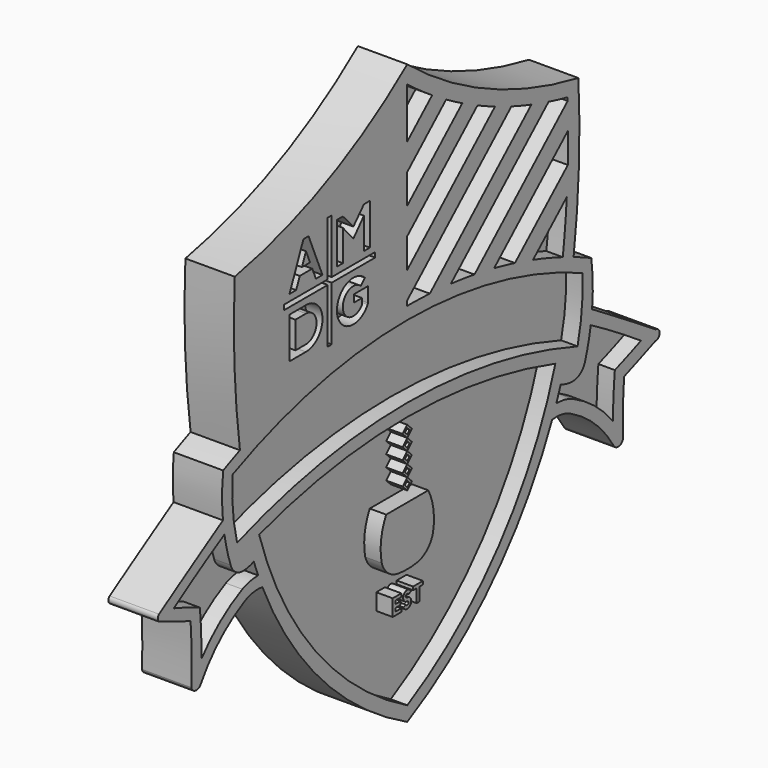
from build123d import *

# Parameters (mm, degrees)
F2_DEPTH = 7.62
F3_DEPTH = 5.08
F4_DEPTH = 7.62


# Not quite as in the source:
# - a feature names something its author has since deleted; it is built from what else it names


with BuildPart() as f2:
    # F0 (on Right) → F2 (new body)
    with BuildSketch(Plane.YZ):
        with BuildLine():
            ThreePointArc((28.5688662104, -6.671875786), (17.7209639174, -26.8909401666), (0, -41.4667758689))
            Line((0, -41.4667758689), (0, -43.7257877909))
            ThreePointArc((0, -43.7257877909), (16.5196456669, -31.2816632656), (27.9511640539, -14.0457903394))
            ThreePointArc((27.9511640539, -14.0457903394), (28.3611811829, -13.0956454783), (28.7550746015, -12.1387038511))
            ThreePointArc((28.7550746015, -12.1387038511), (29.189869611, -11.0251738196), (29.6028329723, -9.9033640792))
            ThreePointArc((29.6028329723, -9.9033640792), (30.0512558711, -8.6014682185), (30.4702761414, -7.2898135606))
            ThreePointArc((30.4702761414, -7.2898135606), (29.5211880551, -6.9758694959), (28.5688662104, -6.671875786))
        make_face()
        with BuildLine():
            ThreePointArc((-29.6028329723, -9.9033640792), (-30.0512558711, -8.6014682185), (-30.4702761414, -7.2898135606))
            ThreePointArc((-30.4702761414, -7.2898135606), (-32.275717496, -7.9177084152), (-34.0682319546, -8.5816077668))
            ThreePointArc((-34.0682319546, -8.5816077668), (-33.1727263346, -9.8516485544), (-31.6970650168, -10.3388421429))
            ThreePointArc((-31.6970650168, -10.3388421429), (-30.6278933435, -10.2271696504), (-29.6028329723, -9.9033640792))
        make_face()
        with BuildLine():
            ThreePointArc((34.3090759298, -8.673933633), (32.3970687067, -7.9613703293), (30.4702761414, -7.2898135606))
            ThreePointArc((30.4702761414, -7.2898135606), (30.0512558711, -8.6014682185), (29.6028329723, -9.9033640792))
            ThreePointArc((29.6028329723, -9.9033640792), (30.7403743709, -10.2999751342), (31.9379090014, -10.4311680127))
            ThreePointArc((31.9379090014, -10.4311680127), (33.4135703165, -9.9439744228), (34.3090759298, -8.673933633))
        make_face()
        with BuildLine():
            ThreePointArc((28.7550746015, -12.1387038511), (28.3611811829, -13.0956454783), (27.9511640539, -14.0457903394))
            ThreePointArc((27.9511640539, -14.0457903394), (29.8035313011, -14.0664319634), (31.5502868159, -14.6833076938))
            ThreePointArc((31.5502868159, -14.6833076938), (36.1922706404, -17.9362667961), (39.7833809257, -22.321889177))
            ThreePointArc((39.7833809257, -22.321889177), (40.7955153713, -22.88098694), (41.6602343321, -22.1133492887))
            ThreePointArc((41.6602343321, -22.1133492887), (41.6260167095, -17.9626931556), (41.8306558255, -13.8169435234))
            ThreePointArc((41.8306558255, -13.8169435234), (44.8619911882, -12.6385051681), (47.8847744868, -11.4383001158))
            ThreePointArc((47.8847744868, -11.4383001158), (48.6831556004, -10.6892682312), (47.9341237159, -9.8908871176))
            ThreePointArc((47.9341237159, -9.8908871176), (41.8140573783, -5.9988864798), (35.658738053, -2.1628827072))
            ThreePointArc((35.658738053, -2.1628827072), (35.5441808227, -3.1869322299), (35.394852187, -4.2064918125))
            ThreePointArc((35.394852187, -4.2064918125), (40.2885281884, -7.1486484466), (45.0794595538, -10.25530696))
            ThreePointArc((45.0794595538, -10.25530696), (42.5737442672, -11.2633717283), (40.041684099, -12.2033052254))
            ThreePointArc((40.041684099, -12.2033052254), (39.7867159057, -15.5987236175), (39.68812496, -19.0022739201))
            ThreePointArc((39.68812496, -19.0022739201), (36.1022922808, -15.4419861489), (31.8168029189, -12.7645945176))
            ThreePointArc((31.8168029189, -12.7645945176), (30.3188612648, -12.2905990682), (28.7550746015, -12.1387038511))
        make_face()
        with BuildLine():
            ThreePointArc((-27.9511640539, -14.0457903394), (-28.3611811829, -13.0956454783), (-28.7550746015, -12.1387038511))
            ThreePointArc((-28.7550746015, -12.1387038511), (-30.3188612648, -12.2905990682), (-31.8168029189, -12.7645945176))
            ThreePointArc((-31.8168029189, -12.7645945176), (-36.1022922808, -15.4419861489), (-39.68812496, -19.0022739201))
            ThreePointArc((-39.68812496, -19.0022739201), (-39.7567496729, -15.4652900802), (-39.9942449201, -11.9356215344))
            ThreePointArc((-39.9942449201, -11.9356215344), (-42.4943140259, -10.9129550124), (-45.0320203748, -9.987623269))
            ThreePointArc((-45.0320203748, -9.987623269), (-40.2016909636, -6.8727936195), (-35.2677039574, -3.9249099398))
            ThreePointArc((-35.2677039574, -3.9249099398), (-35.4270693541, -2.9093430207), (-35.5518756641, -1.8889524672))
            ThreePointArc((-35.5518756641, -1.8889524672), (-41.7369860787, -5.7278399379), (-47.8866845382, -9.6232034266))
            ThreePointArc((-47.8866845382, -9.6232034266), (-48.1257262457, -10.1509293815), (-47.8520728648, -10.6615656987))
            ThreePointArc((-47.8520728648, -10.6615656987), (-44.8292895661, -11.861770751), (-41.7979542035, -13.0402091063))
            ThreePointArc((-41.7979542035, -13.0402091063), (-41.5863132676, -17.5746119455), (-41.6602343321, -22.1133492887))
            ThreePointArc((-41.6602343321, -22.1133492887), (-40.7955153713, -22.88098694), (-39.7833809257, -22.321889177))
            ThreePointArc((-39.7833809257, -22.321889177), (-36.1922706404, -17.9362667961), (-31.5502868159, -14.6833076938))
            ThreePointArc((-31.5502868159, -14.6833076938), (-29.8035313011, -14.0664319634), (-27.9511640539, -14.0457903394))
        make_face()
        with BuildLine():
            ThreePointArc((-28.5688662104, -6.671875786), (-29.5211880551, -6.9758694959), (-30.4702761414, -7.2898135606))
            ThreePointArc((-30.4702761414, -7.2898135606), (-30.0512558711, -8.6014682185), (-29.6028329723, -9.9033640792))
            ThreePointArc((-29.6028329723, -9.9033640792), (-29.189869611, -11.0251738196), (-28.7550746015, -12.1387038511))
            ThreePointArc((-28.7550746015, -12.1387038511), (-28.3611811829, -13.0956454783), (-27.9511640539, -14.0457903394))
            ThreePointArc((-27.9511640539, -14.0457903394), (-16.5196456669, -31.2816632656), (0, -43.7257877909))
            Line((0, -43.7257877909), (0, -41.4667758689))
            ThreePointArc((0, -41.4667758689), (-17.7209639174, -26.8909401666), (-28.5688662104, -6.671875786))
        make_face()
        with BuildLine():
            ThreePointArc((-34.0682319546, -8.5816077668), (-32.275717496, -7.9177084152), (-30.4702761414, -7.2898135606))
            ThreePointArc((-30.4702761414, -7.2898135606), (-29.5211880551, -6.9758694959), (-28.5688662104, -6.671875786))
            ThreePointArc((-28.5688662104, -6.671875786), (0, -2.299220842), (28.5688662104, -6.671875786))
            ThreePointArc((28.5688662104, -6.671875786), (29.5211880551, -6.9758694959), (30.4702761414, -7.2898135606))
            ThreePointArc((30.4702761414, -7.2898135606), (32.3970687067, -7.9613703293), (34.3090759298, -8.673933633))
            ThreePointArc((34.3090759298, -8.673933633), (34.9368600064, -6.4608460088), (35.394852187, -4.2064918125))
            ThreePointArc((35.394852187, -4.2064918125), (35.5441808227, -3.1869322299), (35.658738053, -2.1628827072))
            ThreePointArc((35.658738053, -2.1628827072), (35.7862431554, 1.3568364417), (35.5042511946, 4.8675573039))
            ThreePointArc((35.5042511946, 4.8675573039), (33.8050800577, 5.643593937), (32.088958966, 6.3813905261))
            ThreePointArc((32.088958966, 6.3813905261), (31.0516229156, 6.805512456), (30.008682983, 7.2156609533))
            ThreePointArc((30.008682983, 7.2156609533), (27.1584492935, 8.2553731736), (24.2722940751, 9.1907563256))
            ThreePointArc((24.2722940751, 9.1907563256), (22.5250389094, 9.7013614162), (20.7670586297, 10.1737209285))
            ThreePointArc((20.7670586297, 10.1737209285), (18.7644701082, 10.6621519958), (16.7504251557, 11.100955623))
            ThreePointArc((16.7504251557, 11.100955623), (14.8629765183, 11.4652081673), (12.9676361757, 11.7858750662))
            ThreePointArc((12.9676361757, 11.7858750662), (10.6902549144, 12.1121256668), (8.4047431756, 12.3754523754))
            ThreePointArc((8.4047431756, 12.3754523754), (6.3842218408, 12.5552704602), (4.3599256973, 12.6859078666))
            ThreePointArc((4.3599256973, 12.6859078666), (2.180708045, 12.7714103093), (0, 12.799917618))
            ThreePointArc((0, 12.799917618), (-16.4600536871, 11.15993435), (-32.2729385148, 6.3044646579))
            ThreePointArc((-32.2729385148, 6.3044646579), (-33.8962097721, 5.6031353828), (-35.5042511946, 4.8675573039))
            ThreePointArc((-35.5042511946, 4.8675573039), (-35.7170770288, 1.4906347145), (-35.5518756641, -1.8889524672))
            ThreePointArc((-35.5518756641, -1.8889524672), (-35.4270693541, -2.9093430207), (-35.2677039574, -3.9249099398))
            ThreePointArc((-35.2677039574, -3.9249099398), (-34.7605382134, -6.2771030958), (-34.0682319546, -8.5816077668))
        make_face()
        with BuildLine():
            ThreePointArc((-33.7083284733, 3.5726207659), (-17.2446774523, 9.025399368), (0, 10.8708529679))
            ThreePointArc((0, 10.8708529679), (17.2896098342, 9.0156577322), (33.792024647, 3.5345389662))
            ThreePointArc((33.792024647, 3.5345389662), (33.6890042384, -1.2985833574), (32.8517336285, -6.0597452457))
            ThreePointArc((32.8517336285, -6.0597452457), (0.0193967345, -0.3558691534), (-32.8152080177, -6.0466757012))
            ThreePointArc((-32.8152080177, -6.0466757012), (-33.6517360253, -1.2732347103), (-33.7083284733, 3.5726207659))
        make_face(mode=Mode.SUBTRACT)
        with BuildLine():
            ThreePointArc((-33.2703815176, 30.2840155791), (-33.3383945489, 18.2706664746), (-32.2729385148, 6.3044646579))
            ThreePointArc((-32.2729385148, 6.3044646579), (-16.4600536871, 11.15993435), (0, 12.799917618))
            Line((0, 12.799917618), (0, 13.5470115411))
            Line((0, 13.5470115411), (0, 17.6854213957))
            Line((0, 17.6854213957), (0, 22.2660372864))
            Line((0, 22.2660372864), (0, 26.4044471422))
            Line((0, 26.4044471422), (0, 30.9850630336))
            Line((0, 30.9850630336), (0, 35.123472889))
            Line((0, 35.123472889), (0, 42.8770001444))
            ThreePointArc((0, 42.8770001444), (2.3677216766, 41.1256679461), (4.8004917628, 39.4658787684))
            ThreePointArc((4.8004917628, 39.4658787684), (6.1440586372, 38.6059679212), (7.5050988374, 37.7739894453))
            ThreePointArc((7.5050988374, 37.7739894453), (9.0521255608, 36.8742809791), (10.619583518, 36.0106592104))
            ThreePointArc((10.619583518, 36.0106592104), (12.0755875899, 35.2501172378), (13.5474374931, 34.5207135003))
            ThreePointArc((13.5474374931, 34.5207135003), (15.2251273318, 33.736066262), (16.9211499837, 32.9918743189))
            ThreePointArc((16.9211499837, 32.9918743189), (18.5018678165, 32.3413130995), (20.0965961968, 31.7258944125))
            ThreePointArc((20.0965961968, 31.7258944125), (22.0128328658, 31.0392961839), (23.9464982844, 30.4034360204))
            ThreePointArc((23.9464982844, 30.4034360204), (25.6026977209, 29.9032123795), (27.2696864447, 29.4402125321))
            ThreePointArc((27.2696864447, 29.4402125321), (29.09371693, 28.979244413), (30.9284345114, 28.5628429071))
            ThreePointArc((30.9284345114, 28.5628429071), (30.9390866234, 28.3072147129), (30.94921453, 28.0515652133))
            ThreePointArc((30.94921453, 28.0515652133), (31.0106105135, 26.039411949), (31.0395347413, 24.0265300312))
            ThreePointArc((31.0395347413, 24.0265300312), (31.0323022412, 21.6837727985), (30.9810838152, 19.3415643464))
            ThreePointArc((30.9810838152, 19.3415643464), (30.8960102432, 17.2060844583), (30.7743721396, 15.0723750036))
            ThreePointArc((30.7743721396, 15.0723750036), (30.4536777009, 11.1379610331), (30.008682983, 7.2156609533))
            ThreePointArc((30.008682983, 7.2156609533), (31.0516229156, 6.805512456), (32.088958966, 6.3813905261))
            ThreePointArc((32.088958966, 6.3813905261), (33.1186305942, 18.334974947), (33.0151768056, 30.3323788948))
            ThreePointArc((33.0151768056, 30.3323788948), (15.5682047755, 35.9423036807), (0, 45.6117963866))
            ThreePointArc((0, 45.6117963866), (-15.7054175834, 35.9297463642), (-33.2703815176, 30.2840155791))
        make_face()
        with BuildLine():
            Line((-22.7114348597, 14.4936506769), (-22.7114348597, 20.8402629143))
            Line((-22.7114348597, 20.8402629143), (-19.5476338267, 20.8402629143))
            ThreePointArc((-19.5476338267, 20.8402629143), (-16.3508674463, 17.6669567956), (-19.5476338267, 14.4936506769))
            Line((-19.5476338267, 14.4936506769), (-22.7114348597, 14.4936506769))
        make_face(mode=Mode.SUBTRACT)
        Polygon((-6.189193825, 21.8708057269), (-14.578833418, 21.8708057269), (-14.578833418, 13.4811661339), (-15.3361896718, 13.4811661339), (-15.3361896718, 21.8708057269), (-23.7258292649, 21.8708057269), (-23.7258292649, 22.6281619807), (-15.3361896718, 22.6281619807), (-15.3361896718, 31.0178015738), (-14.578833418, 31.0178015738), (-14.578833418, 22.6281619807), (-6.189193825, 22.6281619807), align=None, mode=Mode.SUBTRACT)
        with BuildLine():
            Line((-8.1508552757, 19.9294396921), (-8.9558750817, 19.1224107936))
            ThreePointArc((-8.9558750817, 19.1224107936), (-12.4318439094, 17.5698783849), (-8.8166163828, 16.3770472559))
            ThreePointArc((-8.8166163828, 16.3770472559), (-8.7538836126, 16.4763115742), (-8.7319527365, 16.5916711946))
            Line((-8.7319527365, 16.5916711946), (-8.7319527365, 17.4191270619))
            Line((-8.7319527365, 17.4191270619), (-10.3048576847, 17.4191270619))
            Line((-10.3048576847, 17.4191270619), (-10.3058647235, 18.5571518939))
            Line((-10.3058647235, 18.5571518939), (-7.5927416105, 18.5595527382))
            Line((-7.5927416105, 18.5595527382), (-7.590726548, 16.2823902296))
            ThreePointArc((-7.590726548, 16.2823902296), (-7.6034442607, 16.178744507), (-7.6410153285, 16.0813145788))
            ThreePointArc((-7.6410153285, 16.0813145788), (-13.5400716848, 17.2575827913), (-8.1508552757, 19.9294396921))
        make_face(mode=Mode.SUBTRACT)
        Polygon((-20.0286190957, 29.9993950033), (-19.0364969938, 29.9993950033), (-16.3545962423, 23.6434713984), (-17.6239740103, 23.6434713984), (-18.3205924604, 25.2944100648), (-20.7354008474, 25.2944100648), (-21.4320192974, 23.6434713984), (-22.7105198472, 23.6434713984), align=None, mode=Mode.SUBTRACT)
        Polygon((-12.4187339097, 28.4452587366), (-12.4187339097, 23.6434713984), (-13.5635240003, 23.6434713984), (-13.5635240003, 29.9993950033), (-12.4187339097, 29.9993950033), (-10.3889470469, 27.789356187), (-8.359160184, 29.9993950033), (-7.2075975113, 29.9993950033), (-7.2075975113, 23.6386322463), (-8.359160184, 23.6386322463), (-8.359160184, 28.4452587366), (-10.3889470469, 26.1637270451), align=None, mode=Mode.SUBTRACT)
        with BuildLine():
            Line((0, 35.123472889), (0, 30.9850630336))
            Line((0, 30.9850630336), (7.5050988374, 37.7739894453))
            ThreePointArc((7.5050988374, 37.7739894453), (6.1440586372, 38.6059679212), (4.8004917628, 39.4658787684))
            Line((4.8004917628, 39.4658787684), (0, 35.123472889))
        make_face()
        with BuildLine():
            Line((0, 26.4044471422), (0, 22.2660372864))
            Line((0, 22.2660372864), (13.5474374931, 34.5207135003))
            ThreePointArc((13.5474374931, 34.5207135003), (12.0755875899, 35.2501172378), (10.619583518, 36.0106592104))
            Line((10.619583518, 36.0106592104), (0, 26.4044471422))
        make_face()
        with BuildLine():
            Line((0, 17.6854213957), (0, 13.5470115411))
            Line((0, 13.5470115411), (20.0965961968, 31.7258944125))
            ThreePointArc((20.0965961968, 31.7258944125), (18.5018678165, 32.3413130995), (16.9211499837, 32.9918743189))
            Line((16.9211499837, 32.9918743189), (0, 17.6854213957))
        make_face()
        with BuildLine():
            Line((23.9464982844, 30.4034360204), (4.3599256973, 12.6859078666))
            ThreePointArc((4.3599256973, 12.6859078666), (6.3842218408, 12.5552704602), (8.4047431756, 12.3754523754))
            Line((8.4047431756, 12.3754523754), (27.2696864447, 29.4402125321))
            ThreePointArc((27.2696864447, 29.4402125321), (25.6026977209, 29.9032123795), (23.9464982844, 30.4034360204))
        make_face()
        with BuildLine():
            Line((30.94921453, 28.0515652133), (12.9676361757, 11.7858750662))
            ThreePointArc((12.9676361757, 11.7858750662), (14.8629765183, 11.4652081673), (16.7504251557, 11.100955623))
            Line((16.7504251557, 11.100955623), (31.0395347413, 24.0265300312))
            ThreePointArc((31.0395347413, 24.0265300312), (31.0106105135, 26.039411949), (30.94921453, 28.0515652133))
        make_face()
        with BuildLine():
            ThreePointArc((20.7670586297, 10.1737209285), (22.5250389094, 9.7013614162), (24.2722940751, 9.1907563256))
            Line((24.2722940751, 9.1907563256), (30.7743721396, 15.0723750036))
            ThreePointArc((30.7743721396, 15.0723750036), (30.8960102432, 17.2060844583), (30.9810838152, 19.3415643464))
            Line((30.9810838152, 19.3415643464), (20.7670586297, 10.1737209285))
        make_face()
    extrude(amount=F2_DEPTH)


with BuildPart() as f2b:
    # F0 (on Right) → F2, piece 2 (new body)
    with BuildSketch(Plane.YZ):
        Polygon((-19.5279966539, 28.1558764371), (-20.3060973907, 26.3118302556), (-18.7498959171, 26.3118302556), align=None)
    extrude(amount=F2_DEPTH)


with BuildPart() as f2c:
    # F0 (on Right) → F2, piece 3 (new body)
    with BuildSketch(Plane.YZ):
        with BuildLine():
            Line((-21.5756800026, 19.6895375848), (-21.5756800026, 15.5159393325))
            Line((-21.5756800026, 15.5159393325), (-19.5476338267, 15.5159393325))
            ThreePointArc((-19.5476338267, 15.5159393325), (-17.4972787499, 17.6027384587), (-19.5476338267, 19.6895375848))
            Line((-19.5476338267, 19.6895375848), (-21.5756800026, 19.6895375848))
        make_face()
    extrude(amount=F2_DEPTH)


with BuildPart() as f3:
    # F0 (on Right) → F3 (new body)
    with BuildSketch(Plane.YZ):
        with BuildLine():
            ThreePointArc((33.792024647, 3.5345389662), (17.2896098342, 9.0156577322), (0, 10.8708529679))
            ThreePointArc((0, 10.8708529679), (-17.2446774523, 9.025399368), (-33.7083284733, 3.5726207659))
            ThreePointArc((-33.7083284733, 3.5726207659), (-33.6517360253, -1.2732347103), (-32.8152080177, -6.0466757012))
            ThreePointArc((-32.8152080177, -6.0466757012), (0.0193967345, -0.3558691534), (32.8517336285, -6.0597452457))
            ThreePointArc((32.8517336285, -6.0597452457), (33.6890042384, -1.2985833574), (33.792024647, 3.5345389662))
        make_face()
    extrude(amount=F3_DEPTH)


with BuildPart() as f3b:
    # F0 (on Right) → F3, piece 2 (new body)
    with BuildSketch(Plane.YZ):
        with BuildLine():
            ThreePointArc((28.5688662104, -6.671875786), (0, -2.299220842), (-28.5688662104, -6.671875786))
            ThreePointArc((-28.5688662104, -6.671875786), (-17.7209639174, -26.8909401666), (0, -41.4667758689))
            ThreePointArc((0, -41.4667758689), (17.7209639174, -26.8909401666), (28.5688662104, -6.671875786))
        make_face()
    extrude(amount=F3_DEPTH)


with BuildPart() as f3c:
    # F0 (on Right) → F3, piece 3 (new body)
    with BuildSketch(Plane.YZ):
        Polygon((-13.5635240003, 23.6434713984), (-12.4187339097, 23.6434713984), (-12.4187339097, 28.4452587366), (-10.3889470469, 26.1637270451), (-8.359160184, 28.4452587366), (-8.359160184, 23.6386322463), (-7.2075975113, 23.6386322463), (-7.2075975113, 29.9993950033), (-8.359160184, 29.9993950033), (-10.3889470469, 27.789356187), (-12.4187339097, 29.9993950033), (-13.5635240003, 29.9993950033), align=None)
    extrude(amount=F3_DEPTH)


with BuildPart() as f3d:
    # F0 (on Right) → F3, piece 4 (new body)
    with BuildSketch(Plane.YZ):
        Polygon((-16.3545962423, 23.6434713984), (-19.0364969938, 29.9993950033), (-20.0286190957, 29.9993950033), (-22.7105198472, 23.6434713984), (-21.4320192974, 23.6434713984), (-20.7354008474, 25.2944100648), (-18.3205924604, 25.2944100648), (-17.6239740103, 23.6434713984), align=None)
        Polygon((-18.7498959171, 26.3118302556), (-20.3060973907, 26.3118302556), (-19.5279966539, 28.1558764371), align=None, mode=Mode.SUBTRACT)
    extrude(amount=F3_DEPTH)


with BuildPart() as f3e:
    # F0 (on Right) → F3, piece 5 (new body)
    with BuildSketch(Plane.YZ):
        with BuildLine():
            Line((-19.5476338267, 20.8402629143), (-22.7114348597, 20.8402629143))
            Line((-22.7114348597, 20.8402629143), (-22.7114348597, 14.4936506769))
            Line((-22.7114348597, 14.4936506769), (-19.5476338267, 14.4936506769))
            ThreePointArc((-19.5476338267, 14.4936506769), (-16.3508674463, 17.6669567956), (-19.5476338267, 20.8402629143))
        make_face()
        with BuildLine():
            Line((-19.5476338267, 15.5159393325), (-21.5756800026, 15.5159393325))
            Line((-21.5756800026, 15.5159393325), (-21.5756800026, 19.6895375848))
            Line((-21.5756800026, 19.6895375848), (-19.5476338267, 19.6895375848))
            ThreePointArc((-19.5476338267, 19.6895375848), (-17.4972787499, 17.6027384587), (-19.5476338267, 15.5159393325))
        make_face(mode=Mode.SUBTRACT)
    extrude(amount=F3_DEPTH)


with BuildPart() as f3f:
    # F0 (on Right) → F3, piece 6 (new body)
    with BuildSketch(Plane.YZ):
        Polygon((-14.578833418, 13.4811661339), (-14.578833418, 21.8708057269), (-6.189193825, 21.8708057269), (-6.189193825, 22.6281619807), (-14.578833418, 22.6281619807), (-14.578833418, 31.0178015738), (-15.3361896718, 31.0178015738), (-15.3361896718, 22.6281619807), (-23.7258292649, 22.6281619807), (-23.7258292649, 21.8708057269), (-15.3361896718, 21.8708057269), (-15.3361896718, 13.4811661339), align=None)
    extrude(amount=F3_DEPTH)


with BuildPart() as f3g:
    # F0 (on Right) → F3, piece 7 (new body)
    with BuildSketch(Plane.YZ):
        with BuildLine():
            ThreePointArc((31.9379090014, -10.4311680127), (30.7403743709, -10.2999751342), (29.6028329723, -9.9033640792))
            ThreePointArc((29.6028329723, -9.9033640792), (29.189869611, -11.0251738196), (28.7550746015, -12.1387038511))
            ThreePointArc((28.7550746015, -12.1387038511), (30.3188612648, -12.2905990682), (31.8168029189, -12.7645945176))
            ThreePointArc((31.8168029189, -12.7645945176), (36.1022922808, -15.4419861489), (39.68812496, -19.0022739201))
            ThreePointArc((39.68812496, -19.0022739201), (39.7867159057, -15.5987236175), (40.041684099, -12.2033052254))
            ThreePointArc((40.041684099, -12.2033052254), (42.5737442672, -11.2633717283), (45.0794595538, -10.25530696))
            ThreePointArc((45.0794595538, -10.25530696), (40.2885281884, -7.1486484466), (35.394852187, -4.2064918125))
            ThreePointArc((35.394852187, -4.2064918125), (34.9368600064, -6.4608460088), (34.3090759298, -8.673933633))
            ThreePointArc((34.3090759298, -8.673933633), (33.4135703165, -9.9439744228), (31.9379090014, -10.4311680127))
        make_face()
    extrude(amount=F3_DEPTH)


with BuildPart() as f3h:
    # F0 (on Right) → F3, piece 8 (new body)
    with BuildSketch(Plane.YZ):
        with BuildLine():
            ThreePointArc((-28.7550746015, -12.1387038511), (-29.189869611, -11.0251738196), (-29.6028329723, -9.9033640792))
            ThreePointArc((-29.6028329723, -9.9033640792), (-30.6278933435, -10.2271696504), (-31.6970650168, -10.3388421429))
            ThreePointArc((-31.6970650168, -10.3388421429), (-33.1727263346, -9.8516485544), (-34.0682319546, -8.5816077668))
            ThreePointArc((-34.0682319546, -8.5816077668), (-34.7605382134, -6.2771030958), (-35.2677039574, -3.9249099398))
            ThreePointArc((-35.2677039574, -3.9249099398), (-40.2016909636, -6.8727936195), (-45.0320203748, -9.987623269))
            ThreePointArc((-45.0320203748, -9.987623269), (-42.4943140259, -10.9129550124), (-39.9942449201, -11.9356215344))
            ThreePointArc((-39.9942449201, -11.9356215344), (-39.7567496729, -15.4652900802), (-39.68812496, -19.0022739201))
            ThreePointArc((-39.68812496, -19.0022739201), (-36.1022922808, -15.4419861489), (-31.8168029189, -12.7645945176))
            ThreePointArc((-31.8168029189, -12.7645945176), (-30.3188612648, -12.2905990682), (-28.7550746015, -12.1387038511))
        make_face()
    extrude(amount=F3_DEPTH)


with BuildPart() as f3i:
    # F0 (on Right) → F3, piece 9 (new body)
    with BuildSketch(Plane.YZ):
        with BuildLine():
            ThreePointArc((-8.8166163828, 16.3770472559), (-12.4318439094, 17.5698783849), (-8.9558750817, 19.1224107936))
            Line((-8.9558750817, 19.1224107936), (-8.1508552757, 19.9294396921))
            ThreePointArc((-8.1508552757, 19.9294396921), (-13.5400716848, 17.2575827913), (-7.6410153285, 16.0813145788))
            ThreePointArc((-7.6410153285, 16.0813145788), (-7.6034442607, 16.178744507), (-7.590726548, 16.2823902296))
            Line((-7.590726548, 16.2823902296), (-7.5927416105, 18.5595527382))
            Line((-7.5927416105, 18.5595527382), (-10.3058647235, 18.5571518939))
            Line((-10.3058647235, 18.5571518939), (-10.3048576847, 17.4191270619))
            Line((-10.3048576847, 17.4191270619), (-8.7319527365, 17.4191270619))
            Line((-8.7319527365, 17.4191270619), (-8.7319527365, 16.5916711946))
            ThreePointArc((-8.7319527365, 16.5916711946), (-8.7538836126, 16.4763115742), (-8.8166163828, 16.3770472559))
        make_face()
    extrude(amount=F3_DEPTH)


with BuildPart() as f3j:
    # F0 (on Right) → F3, piece 10 (new body)
    with BuildSketch(Plane.YZ):
        with BuildLine():
            Line((0, 42.8770001444), (0, 35.123472889))
            Line((0, 35.123472889), (4.8004917628, 39.4658787684))
            ThreePointArc((4.8004917628, 39.4658787684), (2.3677216766, 41.1256679461), (0, 42.8770001444))
        make_face()
    extrude(amount=F3_DEPTH)


with BuildPart() as f3k:
    # F0 (on Right) → F3, piece 11 (new body)
    with BuildSketch(Plane.YZ):
        with BuildLine():
            Line((0, 30.9850630336), (0, 26.4044471422))
            Line((0, 26.4044471422), (10.619583518, 36.0106592104))
            ThreePointArc((10.619583518, 36.0106592104), (9.0521255608, 36.8742809791), (7.5050988374, 37.7739894453))
            Line((7.5050988374, 37.7739894453), (0, 30.9850630336))
        make_face()
    extrude(amount=F3_DEPTH)


with BuildPart() as f3l:
    # F0 (on Right) → F3, piece 12 (new body)
    with BuildSketch(Plane.YZ):
        with BuildLine():
            Line((0, 22.2660372864), (0, 17.6854213957))
            Line((0, 17.6854213957), (16.9211499837, 32.9918743189))
            ThreePointArc((16.9211499837, 32.9918743189), (15.2251273318, 33.736066262), (13.5474374931, 34.5207135003))
            Line((13.5474374931, 34.5207135003), (0, 22.2660372864))
        make_face()
    extrude(amount=F3_DEPTH)


with BuildPart() as f3m:
    # F0 (on Right) → F3, piece 13 (new body)
    with BuildSketch(Plane.YZ):
        with BuildLine():
            Line((0, 13.5470115411), (0, 12.799917618))
            ThreePointArc((0, 12.799917618), (2.180708045, 12.7714103093), (4.3599256973, 12.6859078666))
            Line((4.3599256973, 12.6859078666), (23.9464982844, 30.4034360204))
            ThreePointArc((23.9464982844, 30.4034360204), (22.0128328658, 31.0392961839), (20.0965961968, 31.7258944125))
            Line((20.0965961968, 31.7258944125), (0, 13.5470115411))
        make_face()
    extrude(amount=F3_DEPTH)


with BuildPart() as f3n:
    # F0 (on Right) → F3, piece 14 (new body)
    with BuildSketch(Plane.YZ):
        with BuildLine():
            Line((27.2696864447, 29.4402125321), (8.4047431756, 12.3754523754))
            ThreePointArc((8.4047431756, 12.3754523754), (10.6902549144, 12.1121256668), (12.9676361757, 11.7858750662))
            Line((12.9676361757, 11.7858750662), (30.94921453, 28.0515652133))
            ThreePointArc((30.94921453, 28.0515652133), (30.9390866234, 28.3072147129), (30.9284345114, 28.5628429071))
            ThreePointArc((30.9284345114, 28.5628429071), (29.09371693, 28.979244413), (27.2696864447, 29.4402125321))
        make_face()
    extrude(amount=F3_DEPTH)


with BuildPart() as f3o:
    # F0 (on Right) → F3, piece 15 (new body)
    with BuildSketch(Plane.YZ):
        with BuildLine():
            Line((31.0395347413, 24.0265300312), (16.7504251557, 11.100955623))
            ThreePointArc((16.7504251557, 11.100955623), (18.7644701082, 10.6621519958), (20.7670586297, 10.1737209285))
            Line((20.7670586297, 10.1737209285), (30.9810838152, 19.3415643464))
            ThreePointArc((30.9810838152, 19.3415643464), (31.0323022412, 21.6837727985), (31.0395347413, 24.0265300312))
        make_face()
    extrude(amount=F3_DEPTH)


with BuildPart() as f3p:
    # F0 (on Right) → F3, piece 16 (new body)
    with BuildSketch(Plane.YZ):
        with BuildLine():
            ThreePointArc((24.2722940751, 9.1907563256), (27.1584492935, 8.2553731736), (30.008682983, 7.2156609533))
            ThreePointArc((30.008682983, 7.2156609533), (30.4536777009, 11.1379610331), (30.7743721396, 15.0723750036))
            Line((30.7743721396, 15.0723750036), (24.2722940751, 9.1907563256))
        make_face()
    extrude(amount=F3_DEPTH)


with BuildPart() as f4:
    # F1 (on Right) → F4 (new body)
    with BuildSketch(Plane.YZ):
        Polygon((0.8928787807, -4.2461452918), (0, -3.3532665111), (-0.8928787807, -4.2461452918), (0, -5.1390240725), align=None)
        Polygon((-0.4483685395, -4.2384525274), (0, -3.7900839879), (0.4483685395, -4.2384525274), (0, -4.6868210669), align=None, mode=Mode.SUBTRACT)
    extrude(amount=F4_DEPTH)


with BuildPart() as f4b:
    # F1 (on Right) → F4, piece 2 (new body)
    with BuildSketch(Plane.YZ):
        Polygon((0.8928787807, -6.0319028532), (0, -5.1390240725), (-0.8928787807, -6.0319028532), (0, -6.9247816339), align=None)
        Polygon((0.4483685395, -6.0400648864), (0, -6.4884334259), (-0.4483685395, -6.0400648864), (0, -5.5916963469), align=None, mode=Mode.SUBTRACT)
    extrude(amount=F4_DEPTH)


with BuildPart() as f4c:
    # F1 (on Right) → F4, piece 3 (new body)
    with BuildSketch(Plane.YZ):
        Polygon((0.8928787807, -7.8176604146), (0, -6.9247816339), (-0.8928787807, -7.8176604146), (0, -8.7105391953), align=None)
        Polygon((-0.4483685395, -7.8277371606), (0, -7.3793686211), (0.4483685395, -7.8277371606), (0, -8.2761057001), align=None, mode=Mode.SUBTRACT)
    extrude(amount=F4_DEPTH)


with BuildPart() as f4d:
    # F1 (on Right) → F4, piece 4 (new body)
    with BuildSketch(Plane.YZ):
        Polygon((0.8928787807, -9.603417976), (0, -8.7105391953), (-0.8928787807, -9.603417976), (0, -10.4962967566), align=None)
        Polygon((0.4474029296, -9.6168783493), (-0.0009656099, -10.0652468888), (-0.4493341494, -9.6168783493), (-0.0009656099, -9.1685098098), align=None, mode=Mode.SUBTRACT)
    extrude(amount=F4_DEPTH)


with BuildPart() as f4e:
    # F1 (on Right) → F4, piece 5 (new body)
    with BuildSketch(Plane.YZ):
        Polygon((0.8928787807, -11.3891755373), (0, -10.4962967566), (-0.8928787807, -11.3891755373), (0, -12.282054318), align=None)
        Polygon((-0.4483831412, -11.4074432005), (-1.46017e-05, -10.959074661), (0.4483539378, -11.4074432005), (-1.46017e-05, -11.85581174), align=None, mode=Mode.SUBTRACT)
    extrude(amount=F4_DEPTH)


with BuildPart() as f4f:
    # F1 (on Right) → F4, piece 6 (new body)
    with BuildSketch(Plane.YZ):
        Polygon((-2.2910065018, -26.3003582135), (-1.1374058668, -26.3003582135), (-1.1374058668, -25.7915547118), (-2.8038020246, -25.7915547118), (-2.8038020246, -28.3355722204), (-1.1374058668, -28.3355722204), (-1.1374058668, -27.8267687187), (-2.2910065018, -27.8267687187), (-2.2910065018, -27.3147178814), (-1.2653982267, -27.3147178814), (-1.2653982267, -26.8091617152), (-2.2910065018, -26.8091617152), align=None)
    extrude(amount=F4_DEPTH)


with BuildPart() as f4g:
    # F1 (on Right) → F4, piece 7 (new body)
    with BuildSketch(Plane.YZ):
        Polygon((1.1251628166, -25.7915547118), (1.1251628166, -26.3006044552), (1.8252357914, -26.3006044552), (1.8252357914, -28.3355722204), (2.3306955118, -28.3355722204), (2.3306955118, -26.3006044552), (3.0307684865, -26.3006044552), (3.0307684865, -25.7915547118), align=None)
    extrude(amount=F4_DEPTH)


with BuildPart() as f4h:
    # F1 (on Right) → F4, piece 8 (new body)
    with BuildSketch(Plane.YZ):
        with BuildLine():
            ThreePointArc((-0.0098512966, -27.3424405123), (0.2026423375, -27.7447531682), (-0.2494390903, -27.6934559925))
            Line((-0.2494390903, -27.6934559925), (-0.7286146777, -27.8809393377))
            ThreePointArc((-0.7286146777, -27.8809393377), (0.6276296058, -28.0348308648), (-0.0098512966, -26.8278928972))
            ThreePointArc((-0.0098512966, -26.8278928972), (-0.2230687159, -26.4266463694), (0.2287854472, -26.4744821219))
            Line((0.2287854472, -26.4744821219), (0.7060589349, -26.2822081864))
            ThreePointArc((0.7060589349, -26.2822081864), (-0.6495035546, -26.1387009289), (-0.0098512966, -27.3424405123))
        make_face()
    extrude(amount=F4_DEPTH)


with BuildPart() as f4i:
    # F1 (on Right) → F4, piece 9 (new body)
    with BuildSketch(Plane.YZ):
        with BuildLine():
            Line((4.0624085814, -13.9120751992), (0, -13.9120751992))
            Line((0, -13.9120751992), (-4.0624085814, -13.9120751992))
            ThreePointArc((-4.0624085814, -13.9120751992), (-5.0441458208, -16.948657083), (-4.9295492302, -20.1379368082))
            ThreePointArc((-4.9295492302, -20.1379368082), (-3.8002707254, -21.9136381881), (-1.9072637846, -22.8328280784))
            ThreePointArc((-1.9072637846, -22.8328280784), (0.0087697998, -22.9916870594), (1.9248033842, -22.8328280784))
            ThreePointArc((1.9248033842, -22.8328280784), (3.817810325, -21.9136381881), (4.9470888298, -20.1379368082))
            ThreePointArc((4.9470888298, -20.1379368082), (5.0633176893, -16.9456346687), (4.0624085814, -13.9120751992))
        make_face()
    extrude(amount=F4_DEPTH)


solid = Compound([f2.part, f2b.part, f2c.part, f3.part, f3b.part, f3c.part, f3d.part, f3e.part, f3f.part, f3g.part, f3h.part, f3i.part, f3j.part, f3k.part, f3l.part, f3m.part, f3n.part, f3o.part, f3p.part, f4.part, f4b.part, f4c.part, f4d.part, f4e.part, f4f.part, f4g.part, f4h.part, f4i.part])
